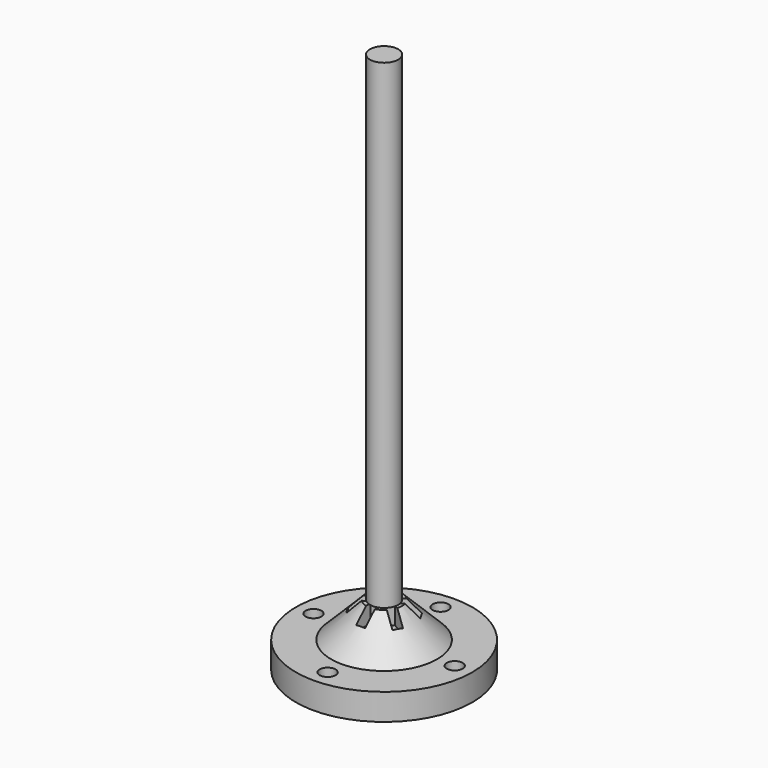
from build123d import *

# Parameters (mm, degrees)
F0_R      = 4
F1_DEPTH  = 136
F2_R      = 15
F3_DEPTH  = 10
F4_SIZE   = 9.99999
F5_R      = 25
F5_R_2    = 15
F6_DEPTH  = 7.5
F7_R      = 2.25
F8_DEPTH  = 153.501
F9_W      = 2.5
F9_H      = 5
F10_DEPTH = 5


# Not quite as in the source:
# - a fillet or chamfer is up to 0.001 mm smaller than in the source, because OpenCascade refuses the exact size


with BuildPart() as f1:
    # F0 (on Top) → F1 (new body)
    with BuildSketch(Plane.XY):
        Circle(F0_R)
    extrude(amount=F1_DEPTH)

    # F2 (on Top) → F3 (join)
    with BuildSketch(Plane.XY):
        Circle(F2_R)
    extrude(amount=-F3_DEPTH)

    # F4 (size 10 in the source; OpenCascade refuses exactly that, so slightly less here)
    f4_edges = [f1.edges().sort_by_distance(p)[0] for p in [
        (-15, 0, 0),
    ]]
    chamfer(f4_edges, length=F4_SIZE)

    # F5 (on face) → F6 (join)
    with BuildSketch(Plane(origin=(0, 0, -10), x_dir=(1, 0, 0), z_dir=(0, 0, -1))):
        Circle(F5_R)
        Circle(F5_R_2, mode=Mode.SUBTRACT)
        Circle(F5_R_2)
    extrude(amount=F6_DEPTH)

    # F7 (on face) → F8 (cut, through all)
    with BuildSketch(Plane(origin=(0, 0, -17.5), x_dir=(1, 0, 0), z_dir=(0, 0, -1))):
        with Locations((-20, 0)):
            Circle(F7_R)
        with Locations((0, 20)):
            Circle(F7_R)
        with Locations((20, 0)):
            Circle(F7_R)
        with Locations((0, -20)):
            Circle(F7_R)
    extrude(amount=-F8_DEPTH, mode=Mode.SUBTRACT)

    # F9 (on face) → F10 (cut)
    with BuildSketch(Plane.XY):
        with Locations((0, 5.8)):
            Rectangle(F9_W, F9_H)
        Polygon((-2.2328838325, 2.7325317547), (-6.5630108514, 5.2325317547), (-7.8130108514, 3.0674682453), (-3.4828838325, 0.5674682453), align=None)
        Polygon((-3.4828838325, -0.5674682453), (-7.8130108514, -3.0674682453), (-6.5630108514, -5.2325317547), (-2.2328838325, -2.7325317547), align=None)
        with Locations((0, -5.8)):
            Rectangle(F9_W, F9_H)
        Polygon((2.2328838325, -2.7325317547), (6.5630108514, -5.2325317547), (7.8130108514, -3.0674682453), (3.4828838325, -0.5674682453), align=None)
        Polygon((3.4828838325, 0.5674682453), (7.8130108514, 3.0674682453), (6.5630108514, 5.2325317547), (2.2328838325, 2.7325317547), align=None)
    extrude(amount=-F10_DEPTH, mode=Mode.SUBTRACT)


solid = f1.part
